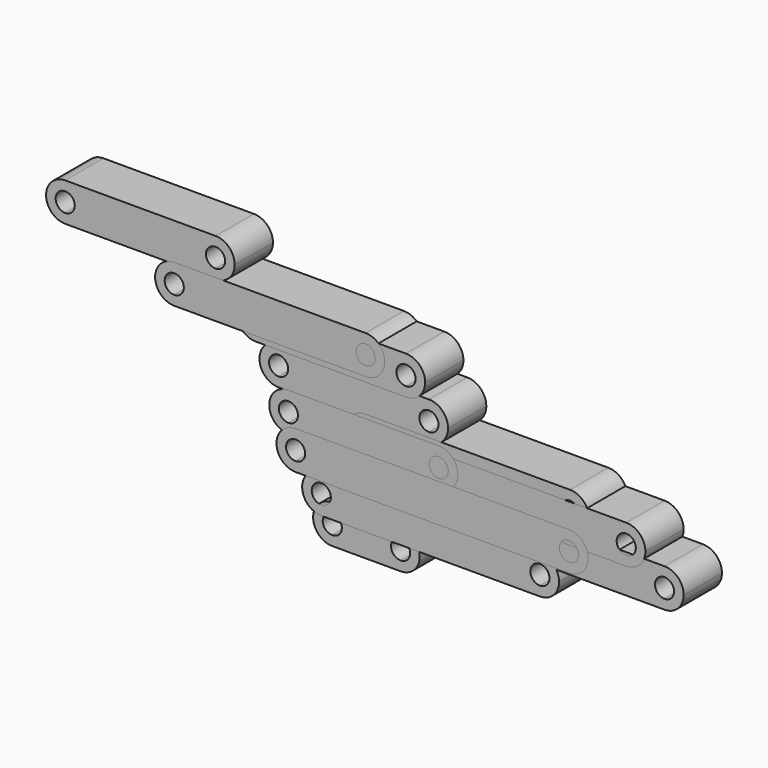
from build123d import *

# Parameters (mm, degrees)
F2_DEPTH  = 6.35
F4_DEPTH  = 6.35
F6_DEPTH  = 6.35
F8_DEPTH  = 6.35
F10_DEPTH = 6.35
F12_DEPTH = 6.35
F14_DEPTH = 6.35
F16_DEPTH = 6.35
F18_DEPTH = 6.35
F20_DEPTH = 6.35
F22_DEPTH = 6.35
F24_DEPTH = 6.35


# Not quite as in the source:
# - a variable given as a bare number and used for a length is read in inches; the dataset says mm whatever the document's units were


with BuildPart() as f2:
    # F1 (on Front) → F2 (new body)
    with BuildSketch(Plane.XZ):
        with BuildLine():
            ThreePointArc((-20.3833308847, 1.27), (-19.4853052726, 0.8980256121), (-19.1133308847, 0))
            ThreePointArc((-19.1133308847, 0), (-19.4853052726, -0.8980256121), (-20.3833308847, -1.27))
            Line((-20.3833308847, -1.27), (-20.3833308847, -2.54))
            ThreePointArc((-20.3833308847, -2.54), (-18.5872796605, -1.7960512242), (-17.8433308847, 0))
            ThreePointArc((-17.8433308847, 0), (-18.5872796605, 1.7960512242), (-20.3833308847, 2.54))
            Line((-20.3833308847, 2.54), (-20.3833308847, 1.27))
        make_face()
        with BuildLine():
            ThreePointArc((-20.3833308847, -1.27), (-21.6533308847, 0), (-20.3833308847, 1.27))
            Line((-20.3833308847, 1.27), (-20.3833308847, 2.54))
            ThreePointArc((-20.3833308847, 2.54), (-22.9233308847, 0), (-20.3833308847, -2.54))
            Line((-20.3833308847, -2.54), (-20.3833308847, -1.27))
        make_face()
        with BuildLine():
            Line((3.202383401, 2.54), (-20.3833308847, 2.54))
            ThreePointArc((-20.3833308847, 2.54), (-18.5872796605, 1.7960512242), (-17.8433308847, 0))
            ThreePointArc((-17.8433308847, 0), (-18.5872796605, -1.7960512242), (-20.3833308847, -2.54))
            Line((-20.3833308847, -2.54), (3.202383401, -2.54))
            ThreePointArc((3.202383401, -2.54), (0.662383401, 0), (3.202383401, 2.54))
        make_face()
        with BuildLine():
            Line((3.202383401, 1.27), (3.202383401, 2.54))
            ThreePointArc((3.202383401, 2.54), (0.662383401, 0), (3.202383401, -2.54))
            Line((3.202383401, -2.54), (3.202383401, -1.27))
            ThreePointArc((3.202383401, -1.27), (1.932383401, 0), (3.202383401, 1.27))
        make_face()
        with BuildLine():
            ThreePointArc((5.742383401, 0), (4.9984346253, 1.7960512242), (3.202383401, 2.54))
            Line((3.202383401, 2.54), (3.202383401, 1.27))
            ThreePointArc((3.202383401, 1.27), (4.1004090131, 0.8980256121), (4.472383401, 0))
            ThreePointArc((4.472383401, 0), (4.1004090131, -0.8980256121), (3.202383401, -1.27))
            Line((3.202383401, -1.27), (3.202383401, -2.54))
            ThreePointArc((3.202383401, -2.54), (4.9984346253, -1.7960512242), (5.742383401, 0))
        make_face()
    extrude(amount=F2_DEPTH)


with BuildPart() as f4:
    # F3 (on Front) → F4 (new body)
    with BuildSketch(Plane.XZ):
        with BuildLine():
            ThreePointArc((-40.9096366516, -5.6361554968), (-40.0116110395, -6.0081298847), (-39.6396366516, -6.9061554968))
            ThreePointArc((-39.6396366516, -6.9061554968), (-40.0116110395, -7.8041811089), (-40.9096366516, -8.1761554968))
            Line((-40.9096366516, -8.1761554968), (-40.9096366516, -9.4461554968))
            ThreePointArc((-40.9096366516, -9.4461554968), (-39.1135854274, -8.702206721), (-38.3696366516, -6.9061554968))
            ThreePointArc((-38.3696366516, -6.9061554968), (-39.1135854274, -5.1101042726), (-40.9096366516, -4.3661554968))
            Line((-40.9096366516, -4.3661554968), (-40.9096366516, -5.6361554968))
        make_face()
        with BuildLine():
            ThreePointArc((-40.9096366516, -8.1761554968), (-42.1796366516, -6.9061554968), (-40.9096366516, -5.6361554968))
            Line((-40.9096366516, -5.6361554968), (-40.9096366516, -4.3661554968))
            ThreePointArc((-40.9096366516, -4.3661554968), (-43.4496366516, -6.9061554968), (-40.9096366516, -9.4461554968))
            Line((-40.9096366516, -9.4461554968), (-40.9096366516, -8.1761554968))
        make_face()
        with BuildLine():
            Line((-31.8382080802, -4.3661554968), (-40.9096366516, -4.3661554968))
            ThreePointArc((-40.9096366516, -4.3661554968), (-39.1135854274, -5.1101042726), (-38.3696366516, -6.9061554968))
            ThreePointArc((-38.3696366516, -6.9061554968), (-39.1135854274, -8.702206721), (-40.9096366516, -9.4461554968))
            Line((-40.9096366516, -9.4461554968), (-31.8382080802, -9.4461554968))
            ThreePointArc((-31.8382080802, -9.4461554968), (-34.3782080802, -6.9061554968), (-31.8382080802, -4.3661554968))
        make_face()
        with BuildLine():
            Line((-31.8382080802, -5.6361554968), (-31.8382080802, -4.3661554968))
            ThreePointArc((-31.8382080802, -4.3661554968), (-34.3782080802, -6.9061554968), (-31.8382080802, -9.4461554968))
            Line((-31.8382080802, -9.4461554968), (-31.8382080802, -8.1761554968))
            ThreePointArc((-31.8382080802, -8.1761554968), (-33.1082080802, -6.9061554968), (-31.8382080802, -5.6361554968))
        make_face()
        with BuildLine():
            ThreePointArc((-29.2982080802, -6.9061554968), (-30.042156856, -5.1101042726), (-31.8382080802, -4.3661554968))
            Line((-31.8382080802, -4.3661554968), (-31.8382080802, -5.6361554968))
            ThreePointArc((-31.8382080802, -5.6361554968), (-30.9401824681, -6.0081298847), (-30.5682080802, -6.9061554968))
            ThreePointArc((-30.5682080802, -6.9061554968), (-30.9401824681, -7.8041811089), (-31.8382080802, -8.1761554968))
            Line((-31.8382080802, -8.1761554968), (-31.8382080802, -9.4461554968))
            ThreePointArc((-31.8382080802, -9.4461554968), (-30.042156856, -8.702206721), (-29.2982080802, -6.9061554968))
        make_face()
    extrude(amount=F4_DEPTH)


with BuildPart() as f6:
    # F5 (on Front) → F6 (new body)
    with BuildSketch(Plane.XZ):
        with BuildLine():
            ThreePointArc((-42.3683448485, -2.56121497), (-41.4703192364, -2.9331893579), (-41.0983448485, -3.83121497))
            ThreePointArc((-41.0983448485, -3.83121497), (-41.4703192364, -4.7292405821), (-42.3683448485, -5.10121497))
            Line((-42.3683448485, -5.10121497), (-42.3683448485, -6.37121497))
            ThreePointArc((-42.3683448485, -6.37121497), (-40.5722936243, -5.6272661942), (-39.8283448485, -3.83121497))
            ThreePointArc((-39.8283448485, -3.83121497), (-40.5722936243, -2.0351637458), (-42.3683448485, -1.29121497))
            Line((-42.3683448485, -1.29121497), (-42.3683448485, -2.56121497))
        make_face()
        with BuildLine():
            ThreePointArc((-42.3683448485, -5.10121497), (-43.6383448485, -3.83121497), (-42.3683448485, -2.56121497))
            Line((-42.3683448485, -2.56121497), (-42.3683448485, -1.29121497))
            ThreePointArc((-42.3683448485, -1.29121497), (-44.9083448485, -3.83121497), (-42.3683448485, -6.37121497))
            Line((-42.3683448485, -6.37121497), (-42.3683448485, -5.10121497))
        make_face()
        with BuildLine():
            Line((-13.3397734199, -1.29121497), (-42.3683448485, -1.29121497))
            ThreePointArc((-42.3683448485, -1.29121497), (-40.5722936243, -2.0351637458), (-39.8283448485, -3.83121497))
            ThreePointArc((-39.8283448485, -3.83121497), (-40.5722936243, -5.6272661942), (-42.3683448485, -6.37121497))
            Line((-42.3683448485, -6.37121497), (-13.3397734199, -6.37121497))
            ThreePointArc((-13.3397734199, -6.37121497), (-15.8797734199, -3.83121497), (-13.3397734199, -1.29121497))
        make_face()
        with BuildLine():
            Line((-13.3397734199, -2.56121497), (-13.3397734199, -1.29121497))
            ThreePointArc((-13.3397734199, -1.29121497), (-15.8797734199, -3.83121497), (-13.3397734199, -6.37121497))
            Line((-13.3397734199, -6.37121497), (-13.3397734199, -5.10121497))
            ThreePointArc((-13.3397734199, -5.10121497), (-14.6097734199, -3.83121497), (-13.3397734199, -2.56121497))
        make_face()
        with BuildLine():
            ThreePointArc((-10.7997734199, -3.83121497), (-11.5437221957, -2.0351637458), (-13.3397734199, -1.29121497))
            Line((-13.3397734199, -1.29121497), (-13.3397734199, -2.56121497))
            ThreePointArc((-13.3397734199, -2.56121497), (-12.4417478078, -2.9331893579), (-12.0697734199, -3.83121497))
            ThreePointArc((-12.0697734199, -3.83121497), (-12.4417478078, -4.7292405821), (-13.3397734199, -5.10121497))
            Line((-13.3397734199, -5.10121497), (-13.3397734199, -6.37121497))
            ThreePointArc((-13.3397734199, -6.37121497), (-11.5437221957, -5.6272661942), (-10.7997734199, -3.83121497))
        make_face()
    extrude(amount=F6_DEPTH)


with BuildPart() as f8:
    # F7 (on Front) → F8 (new body)
    with BuildSketch(Plane.XZ):
        with BuildLine():
            ThreePointArc((-48.0340662203, 10.5945822936), (-47.1360406082, 10.2226079057), (-46.7640662203, 9.3245822936))
            ThreePointArc((-46.7640662203, 9.3245822936), (-47.1360406082, 8.4265566815), (-48.0340662203, 8.0545822936))
            Line((-48.0340662203, 8.0545822936), (-48.0340662203, 6.7845822936))
            ThreePointArc((-48.0340662203, 6.7845822936), (-46.2380149961, 7.5285310694), (-45.4940662203, 9.3245822936))
            ThreePointArc((-45.4940662203, 9.3245822936), (-46.2380149961, 11.1206335178), (-48.0340662203, 11.8645822936))
            Line((-48.0340662203, 11.8645822936), (-48.0340662203, 10.5945822936))
        make_face()
        with BuildLine():
            ThreePointArc((-48.0340662203, 8.0545822936), (-49.3040662203, 9.3245822936), (-48.0340662203, 10.5945822936))
            Line((-48.0340662203, 10.5945822936), (-48.0340662203, 11.8645822936))
            ThreePointArc((-48.0340662203, 11.8645822936), (-50.5740662203, 9.3245822936), (-48.0340662203, 6.7845822936))
            Line((-48.0340662203, 6.7845822936), (-48.0340662203, 8.0545822936))
        make_face()
        with BuildLine():
            Line((-28.0769233631, 11.8645822936), (-48.0340662203, 11.8645822936))
            ThreePointArc((-48.0340662203, 11.8645822936), (-46.2380149961, 11.1206335178), (-45.4940662203, 9.3245822936))
            ThreePointArc((-45.4940662203, 9.3245822936), (-46.2380149961, 7.5285310694), (-48.0340662203, 6.7845822936))
            Line((-48.0340662203, 6.7845822936), (-28.0769233631, 6.7845822936))
            ThreePointArc((-28.0769233631, 6.7845822936), (-30.6169233631, 9.3245822936), (-28.0769233631, 11.8645822936))
        make_face()
        with BuildLine():
            Line((-28.0769233631, 10.5945822936), (-28.0769233631, 11.8645822936))
            ThreePointArc((-28.0769233631, 11.8645822936), (-30.6169233631, 9.3245822936), (-28.0769233631, 6.7845822936))
            Line((-28.0769233631, 6.7845822936), (-28.0769233631, 8.0545822936))
            ThreePointArc((-28.0769233631, 8.0545822936), (-29.3469233631, 9.3245822936), (-28.0769233631, 10.5945822936))
        make_face()
        with BuildLine():
            ThreePointArc((-25.5369233631, 9.3245822936), (-26.2808721389, 11.1206335178), (-28.0769233631, 11.8645822936))
            Line((-28.0769233631, 11.8645822936), (-28.0769233631, 10.5945822936))
            ThreePointArc((-28.0769233631, 10.5945822936), (-27.178897751, 10.2226079057), (-26.8069233631, 9.3245822936))
            ThreePointArc((-26.8069233631, 9.3245822936), (-27.178897751, 8.4265566815), (-28.0769233631, 8.0545822936))
            Line((-28.0769233631, 8.0545822936), (-28.0769233631, 6.7845822936))
            ThreePointArc((-28.0769233631, 6.7845822936), (-26.2808721389, 7.5285310694), (-25.5369233631, 9.3245822936))
        make_face()
    extrude(amount=F8_DEPTH)


with BuildPart() as f10:
    # F9 (on Front) → F10 (new body)
    with BuildSketch(Plane.XZ):
        with BuildLine():
            ThreePointArc((-38.6977585754, 1.7656836929), (-37.7997329633, 1.393709305), (-37.4277585754, 0.4956836929))
            ThreePointArc((-37.4277585754, 0.4956836929), (-37.7997329633, -0.4023419192), (-38.6977585754, -0.7743163071))
            Line((-38.6977585754, -0.7743163071), (-38.6977585754, -2.0443163071))
            ThreePointArc((-38.6977585754, -2.0443163071), (-36.9017073512, -1.3003675314), (-36.1577585754, 0.4956836929))
            ThreePointArc((-36.1577585754, 0.4956836929), (-36.9017073512, 2.2917349171), (-38.6977585754, 3.0356836929))
            Line((-38.6977585754, 3.0356836929), (-38.6977585754, 1.7656836929))
        make_face()
        with BuildLine():
            ThreePointArc((-38.6977585754, -0.7743163071), (-39.9677585754, 0.4956836929), (-38.6977585754, 1.7656836929))
            Line((-38.6977585754, 1.7656836929), (-38.6977585754, 3.0356836929))
            ThreePointArc((-38.6977585754, 3.0356836929), (-41.2377585754, 0.4956836929), (-38.6977585754, -2.0443163071))
            Line((-38.6977585754, -2.0443163071), (-38.6977585754, -0.7743163071))
        make_face()
        with BuildLine():
            Line((-18.7406157183, 3.0356836929), (-38.6977585754, 3.0356836929))
            ThreePointArc((-38.6977585754, 3.0356836929), (-36.9017073512, 2.2917349171), (-36.1577585754, 0.4956836929))
            ThreePointArc((-36.1577585754, 0.4956836929), (-36.9017073512, -1.3003675314), (-38.6977585754, -2.0443163071))
            Line((-38.6977585754, -2.0443163071), (-18.7406157183, -2.0443163071))
            ThreePointArc((-18.7406157183, -2.0443163071), (-21.2806157183, 0.4956836929), (-18.7406157183, 3.0356836929))
        make_face()
        with BuildLine():
            Line((-18.7406157183, 1.7656836929), (-18.7406157183, 3.0356836929))
            ThreePointArc((-18.7406157183, 3.0356836929), (-21.2806157183, 0.4956836929), (-18.7406157183, -2.0443163071))
            Line((-18.7406157183, -2.0443163071), (-18.7406157183, -0.7743163071))
            ThreePointArc((-18.7406157183, -0.7743163071), (-20.0106157183, 0.4956836929), (-18.7406157183, 1.7656836929))
        make_face()
        with BuildLine():
            ThreePointArc((-16.2006157183, 0.4956836929), (-16.9445644941, 2.2917349171), (-18.7406157183, 3.0356836929))
            Line((-18.7406157183, 3.0356836929), (-18.7406157183, 1.7656836929))
            ThreePointArc((-18.7406157183, 1.7656836929), (-17.8425901062, 1.393709305), (-17.4706157183, 0.4956836929))
            ThreePointArc((-17.4706157183, 0.4956836929), (-17.8425901062, -0.4023419192), (-18.7406157183, -0.7743163071))
            Line((-18.7406157183, -0.7743163071), (-18.7406157183, -2.0443163071))
            ThreePointArc((-18.7406157183, -2.0443163071), (-16.9445644941, -1.3003675314), (-16.2006157183, 0.4956836929))
        make_face()
    extrude(amount=F10_DEPTH)


with BuildPart() as f12:
    # F11 (on Front) → F12 (new body)
    with BuildSketch(Plane.XZ):
        with BuildLine():
            ThreePointArc((-36.5666438616, 6.1293925312), (-35.6686182495, 5.7574181433), (-35.2966438616, 4.8593925312))
            ThreePointArc((-35.2966438616, 4.8593925312), (-35.6686182495, 3.9613669191), (-36.5666438616, 3.5893925312))
            Line((-36.5666438616, 3.5893925312), (-36.5666438616, 2.3193925312))
            ThreePointArc((-36.5666438616, 2.3193925312), (-34.7705926374, 3.063341307), (-34.0266438616, 4.8593925312))
            ThreePointArc((-34.0266438616, 4.8593925312), (-34.7705926374, 6.6554437554), (-36.5666438616, 7.3993925312))
            Line((-36.5666438616, 7.3993925312), (-36.5666438616, 6.1293925312))
        make_face()
        with BuildLine():
            ThreePointArc((-36.5666438616, 3.5893925312), (-37.8366438616, 4.8593925312), (-36.5666438616, 6.1293925312))
            Line((-36.5666438616, 6.1293925312), (-36.5666438616, 7.3993925312))
            ThreePointArc((-36.5666438616, 7.3993925312), (-39.1066438616, 4.8593925312), (-36.5666438616, 2.3193925312))
            Line((-36.5666438616, 2.3193925312), (-36.5666438616, 3.5893925312))
        make_face()
        with BuildLine():
            Line((-9.3523581473, 7.3993925312), (-36.5666438616, 7.3993925312))
            ThreePointArc((-36.5666438616, 7.3993925312), (-34.7705926374, 6.6554437554), (-34.0266438616, 4.8593925312))
            ThreePointArc((-34.0266438616, 4.8593925312), (-34.7705926374, 3.063341307), (-36.5666438616, 2.3193925312))
            Line((-36.5666438616, 2.3193925312), (-9.3523581473, 2.3193925312))
            ThreePointArc((-9.3523581473, 2.3193925312), (-11.8923581473, 4.8593925312), (-9.3523581473, 7.3993925312))
        make_face()
        with BuildLine():
            Line((-9.3523581473, 6.1293925312), (-9.3523581473, 7.3993925312))
            ThreePointArc((-9.3523581473, 7.3993925312), (-11.8923581473, 4.8593925312), (-9.3523581473, 2.3193925312))
            Line((-9.3523581473, 2.3193925312), (-9.3523581473, 3.5893925312))
            ThreePointArc((-9.3523581473, 3.5893925312), (-10.6223581473, 4.8593925312), (-9.3523581473, 6.1293925312))
        make_face()
        with BuildLine():
            ThreePointArc((-6.8123581473, 4.8593925312), (-7.5563069231, 6.6554437554), (-9.3523581473, 7.3993925312))
            Line((-9.3523581473, 7.3993925312), (-9.3523581473, 6.1293925312))
            ThreePointArc((-9.3523581473, 6.1293925312), (-8.4543325352, 5.7574181433), (-8.0823581473, 4.8593925312))
            ThreePointArc((-8.0823581473, 4.8593925312), (-8.4543325352, 3.9613669191), (-9.3523581473, 3.5893925312))
            Line((-9.3523581473, 3.5893925312), (-9.3523581473, 2.3193925312))
            ThreePointArc((-9.3523581473, 2.3193925312), (-7.5563069231, 3.063341307), (-6.8123581473, 4.8593925312))
        make_face()
    extrude(amount=F12_DEPTH)


with BuildPart() as f14:
    # F13 (on Front) → F14 (new body)
    with BuildSketch(Plane.XZ):
        with BuildLine():
            ThreePointArc((-34.5370125747, 4.7086499319), (-33.6389869626, 4.336675544), (-33.2670125747, 3.4386499319))
            ThreePointArc((-33.2670125747, 3.4386499319), (-33.6389869626, 2.5406243198), (-34.5370125747, 2.1686499319))
            Line((-34.5370125747, 2.1686499319), (-34.5370125747, 0.8986499319))
            ThreePointArc((-34.5370125747, 0.8986499319), (-32.7409613505, 1.6425987077), (-31.9970125747, 3.4386499319))
            ThreePointArc((-31.9970125747, 3.4386499319), (-32.7409613505, 5.2347011561), (-34.5370125747, 5.9786499319))
            Line((-34.5370125747, 5.9786499319), (-34.5370125747, 4.7086499319))
        make_face()
        with BuildLine():
            ThreePointArc((-34.5370125747, 2.1686499319), (-35.8070125747, 3.4386499319), (-34.5370125747, 4.7086499319))
            Line((-34.5370125747, 4.7086499319), (-34.5370125747, 5.9786499319))
            ThreePointArc((-34.5370125747, 5.9786499319), (-37.0770125747, 3.4386499319), (-34.5370125747, 0.8986499319))
            Line((-34.5370125747, 0.8986499319), (-34.5370125747, 2.1686499319))
        make_face()
        with BuildLine():
            Line((-1.8798697176, 5.9786499319), (-34.5370125747, 5.9786499319))
            ThreePointArc((-34.5370125747, 5.9786499319), (-32.7409613505, 5.2347011561), (-31.9970125747, 3.4386499319))
            ThreePointArc((-31.9970125747, 3.4386499319), (-32.7409613505, 1.6425987077), (-34.5370125747, 0.8986499319))
            Line((-34.5370125747, 0.8986499319), (-1.8798697176, 0.8986499319))
            ThreePointArc((-1.8798697176, 0.8986499319), (-4.4198697176, 3.4386499319), (-1.8798697176, 5.9786499319))
        make_face()
        with BuildLine():
            Line((-1.8798697176, 4.7086499319), (-1.8798697176, 5.9786499319))
            ThreePointArc((-1.8798697176, 5.9786499319), (-4.4198697176, 3.4386499319), (-1.8798697176, 0.8986499319))
            Line((-1.8798697176, 0.8986499319), (-1.8798697176, 2.1686499319))
            ThreePointArc((-1.8798697176, 2.1686499319), (-3.1498697176, 3.4386499319), (-1.8798697176, 4.7086499319))
        make_face()
        with BuildLine():
            ThreePointArc((0.6601302824, 3.4386499319), (-0.0838184934, 5.2347011561), (-1.8798697176, 5.9786499319))
            Line((-1.8798697176, 5.9786499319), (-1.8798697176, 4.7086499319))
            ThreePointArc((-1.8798697176, 4.7086499319), (-0.9818441055, 4.336675544), (-0.6098697176, 3.4386499319))
            ThreePointArc((-0.6098697176, 3.4386499319), (-0.9818441055, 2.5406243198), (-1.8798697176, 2.1686499319))
            Line((-1.8798697176, 2.1686499319), (-1.8798697176, 0.8986499319))
            ThreePointArc((-1.8798697176, 0.8986499319), (-0.0838184934, 1.6425987077), (0.6601302824, 3.4386499319))
        make_face()
    extrude(amount=F14_DEPTH)


with BuildPart() as f16:
    # F15 (on Front) → F16 (new body)
    with BuildSketch(Plane.XZ):
        with BuildLine():
            ThreePointArc((-51.0785131506, 14.958291423), (-50.1804875384, 14.5863170351), (-49.8085131506, 13.688291423))
            ThreePointArc((-49.8085131506, 13.688291423), (-50.1804875384, 12.7902658109), (-51.0785131506, 12.418291423))
            Line((-51.0785131506, 12.418291423), (-51.0785131506, 11.148291423))
            ThreePointArc((-51.0785131506, 11.148291423), (-49.2824619263, 11.8922401988), (-48.5385131506, 13.688291423))
            ThreePointArc((-48.5385131506, 13.688291423), (-49.2824619263, 15.4843426472), (-51.0785131506, 16.228291423))
            Line((-51.0785131506, 16.228291423), (-51.0785131506, 14.958291423))
        make_face()
        with BuildLine():
            ThreePointArc((-51.0785131506, 12.418291423), (-52.3485131506, 13.688291423), (-51.0785131506, 14.958291423))
            Line((-51.0785131506, 14.958291423), (-51.0785131506, 16.228291423))
            ThreePointArc((-51.0785131506, 16.228291423), (-53.6185131506, 13.688291423), (-51.0785131506, 11.148291423))
            Line((-51.0785131506, 11.148291423), (-51.0785131506, 12.418291423))
        make_face()
        with BuildLine():
            Line((-31.1213702934, 16.228291423), (-51.0785131506, 16.228291423))
            ThreePointArc((-51.0785131506, 16.228291423), (-49.2824619263, 15.4843426472), (-48.5385131506, 13.688291423))
            ThreePointArc((-48.5385131506, 13.688291423), (-49.2824619263, 11.8922401988), (-51.0785131506, 11.148291423))
            Line((-51.0785131506, 11.148291423), (-31.1213702934, 11.148291423))
            ThreePointArc((-31.1213702934, 11.148291423), (-33.6613702934, 13.688291423), (-31.1213702934, 16.228291423))
        make_face()
        with BuildLine():
            Line((-31.1213702934, 14.958291423), (-31.1213702934, 16.228291423))
            ThreePointArc((-31.1213702934, 16.228291423), (-33.6613702934, 13.688291423), (-31.1213702934, 11.148291423))
            Line((-31.1213702934, 11.148291423), (-31.1213702934, 12.418291423))
            ThreePointArc((-31.1213702934, 12.418291423), (-32.3913702934, 13.688291423), (-31.1213702934, 14.958291423))
        make_face()
        with BuildLine():
            ThreePointArc((-28.5813702934, 13.688291423), (-29.3253190692, 15.4843426472), (-31.1213702934, 16.228291423))
            Line((-31.1213702934, 16.228291423), (-31.1213702934, 14.958291423))
            ThreePointArc((-31.1213702934, 14.958291423), (-30.2233446813, 14.5863170351), (-29.8513702934, 13.688291423))
            ThreePointArc((-29.8513702934, 13.688291423), (-30.2233446813, 12.7902658109), (-31.1213702934, 12.418291423))
            Line((-31.1213702934, 12.418291423), (-31.1213702934, 11.148291423))
            ThreePointArc((-31.1213702934, 11.148291423), (-29.3253190692, 11.8922401988), (-28.5813702934, 13.688291423))
        make_face()
    extrude(amount=F16_DEPTH)


with BuildPart() as f18:
    # F17 (on Front) → F18 (new body)
    with BuildSketch(Plane.XZ):
        with BuildLine():
            ThreePointArc((-76.3660705439, 20.4931088877), (-75.4680449318, 20.1211344998), (-75.0960705439, 19.2231088877))
            ThreePointArc((-75.0960705439, 19.2231088877), (-75.4680449318, 18.3250832756), (-76.3660705439, 17.9531088877))
            Line((-76.3660705439, 17.9531088877), (-76.3660705439, 16.6831088877))
            ThreePointArc((-76.3660705439, 16.6831088877), (-74.5700193197, 17.4270576635), (-73.8260705439, 19.2231088877))
            ThreePointArc((-73.8260705439, 19.2231088877), (-74.5700193197, 21.0191601119), (-76.3660705439, 21.7631088877))
            Line((-76.3660705439, 21.7631088877), (-76.3660705439, 20.4931088877))
        make_face()
        with BuildLine():
            ThreePointArc((-76.3660705439, 17.9531088877), (-77.6360705439, 19.2231088877), (-76.3660705439, 20.4931088877))
            Line((-76.3660705439, 20.4931088877), (-76.3660705439, 21.7631088877))
            ThreePointArc((-76.3660705439, 21.7631088877), (-78.9060705439, 19.2231088877), (-76.3660705439, 16.6831088877))
            Line((-76.3660705439, 16.6831088877), (-76.3660705439, 17.9531088877))
        make_face()
        with BuildLine():
            Line((-56.4089276867, 21.7631088877), (-76.3660705439, 21.7631088877))
            ThreePointArc((-76.3660705439, 21.7631088877), (-74.5700193197, 21.0191601119), (-73.8260705439, 19.2231088877))
            ThreePointArc((-73.8260705439, 19.2231088877), (-74.5700193197, 17.4270576635), (-76.3660705439, 16.6831088877))
            Line((-76.3660705439, 16.6831088877), (-56.4089276867, 16.6831088877))
            ThreePointArc((-56.4089276867, 16.6831088877), (-58.9489276867, 19.2231088877), (-56.4089276867, 21.7631088877))
        make_face()
        with BuildLine():
            Line((-56.4089276867, 20.4931088877), (-56.4089276867, 21.7631088877))
            ThreePointArc((-56.4089276867, 21.7631088877), (-58.9489276867, 19.2231088877), (-56.4089276867, 16.6831088877))
            Line((-56.4089276867, 16.6831088877), (-56.4089276867, 17.9531088877))
            ThreePointArc((-56.4089276867, 17.9531088877), (-57.6789276867, 19.2231088877), (-56.4089276867, 20.4931088877))
        make_face()
        with BuildLine():
            ThreePointArc((-53.8689276867, 19.2231088877), (-54.6128764625, 21.0191601119), (-56.4089276867, 21.7631088877))
            Line((-56.4089276867, 21.7631088877), (-56.4089276867, 20.4931088877))
            ThreePointArc((-56.4089276867, 20.4931088877), (-55.5109020746, 20.1211344998), (-55.1389276867, 19.2231088877))
            ThreePointArc((-55.1389276867, 19.2231088877), (-55.5109020746, 18.3250832756), (-56.4089276867, 17.9531088877))
            Line((-56.4089276867, 17.9531088877), (-56.4089276867, 16.6831088877))
            ThreePointArc((-56.4089276867, 16.6831088877), (-54.6128764625, 17.4270576635), (-53.8689276867, 19.2231088877))
        make_face()
    extrude(amount=F18_DEPTH)


with BuildPart() as f20:
    # F19 (on Front) → F20 (new body)
    with BuildSketch(Plane.XZ):
        with BuildLine():
            ThreePointArc((-46.7356982431, 5.5978406374), (-45.837672631, 5.2258662495), (-45.4656982431, 4.3278406374))
            ThreePointArc((-45.4656982431, 4.3278406374), (-45.837672631, 3.4298150253), (-46.7356982431, 3.0578406374))
            Line((-46.7356982431, 3.0578406374), (-46.7356982431, 1.7878406374))
            ThreePointArc((-46.7356982431, 1.7878406374), (-44.9396470189, 2.5317894132), (-44.1956982431, 4.3278406374))
            ThreePointArc((-44.1956982431, 4.3278406374), (-44.9396470189, 6.1238918616), (-46.7356982431, 6.8678406374))
            Line((-46.7356982431, 6.8678406374), (-46.7356982431, 5.5978406374))
        make_face()
        with BuildLine():
            ThreePointArc((-46.7356982431, 3.0578406374), (-48.0056982431, 4.3278406374), (-46.7356982431, 5.5978406374))
            Line((-46.7356982431, 5.5978406374), (-46.7356982431, 6.8678406374))
            ThreePointArc((-46.7356982431, 6.8678406374), (-49.2756982431, 4.3278406374), (-46.7356982431, 1.7878406374))
            Line((-46.7356982431, 1.7878406374), (-46.7356982431, 3.0578406374))
        make_face()
        with BuildLine():
            Line((-26.778555386, 6.8678406374), (-46.7356982431, 6.8678406374))
            ThreePointArc((-46.7356982431, 6.8678406374), (-44.9396470189, 6.1238918616), (-44.1956982431, 4.3278406374))
            ThreePointArc((-44.1956982431, 4.3278406374), (-44.9396470189, 2.5317894132), (-46.7356982431, 1.7878406374))
            Line((-46.7356982431, 1.7878406374), (-26.778555386, 1.7878406374))
            ThreePointArc((-26.778555386, 1.7878406374), (-29.318555386, 4.3278406374), (-26.778555386, 6.8678406374))
        make_face()
        with BuildLine():
            Line((-26.778555386, 5.5978406374), (-26.778555386, 6.8678406374))
            ThreePointArc((-26.778555386, 6.8678406374), (-29.318555386, 4.3278406374), (-26.778555386, 1.7878406374))
            Line((-26.778555386, 1.7878406374), (-26.778555386, 3.0578406374))
            ThreePointArc((-26.778555386, 3.0578406374), (-28.048555386, 4.3278406374), (-26.778555386, 5.5978406374))
        make_face()
        with BuildLine():
            ThreePointArc((-24.238555386, 4.3278406374), (-24.9825041618, 6.1238918616), (-26.778555386, 6.8678406374))
            Line((-26.778555386, 6.8678406374), (-26.778555386, 5.5978406374))
            ThreePointArc((-26.778555386, 5.5978406374), (-25.8805297739, 5.2258662495), (-25.508555386, 4.3278406374))
            ThreePointArc((-25.508555386, 4.3278406374), (-25.8805297739, 3.4298150253), (-26.778555386, 3.0578406374))
            Line((-26.778555386, 3.0578406374), (-26.778555386, 1.7878406374))
            ThreePointArc((-26.778555386, 1.7878406374), (-24.9825041618, 2.5317894132), (-24.238555386, 4.3278406374))
        make_face()
    extrude(amount=F20_DEPTH)


with BuildPart() as f22:
    # F21 (on Front) → F22 (new body)
    with BuildSketch(Plane.XZ):
        with BuildLine():
            ThreePointArc((-45.7747111819, 1.4335720691), (-44.8766855698, 1.0615976812), (-44.5047111819, 0.1635720691))
            ThreePointArc((-44.5047111819, 0.1635720691), (-44.8766855698, -0.734453543), (-45.7747111819, -1.1064279309))
            Line((-45.7747111819, -1.1064279309), (-45.7747111819, -2.3764279309))
            ThreePointArc((-45.7747111819, -2.3764279309), (-43.9786599576, -1.6324791551), (-43.2347111819, 0.1635720691))
            ThreePointArc((-43.2347111819, 0.1635720691), (-43.9786599576, 1.9596232934), (-45.7747111819, 2.7035720691))
            Line((-45.7747111819, 2.7035720691), (-45.7747111819, 1.4335720691))
        make_face()
        with BuildLine():
            ThreePointArc((-45.7747111819, -1.1064279309), (-47.0447111819, 0.1635720691), (-45.7747111819, 1.4335720691))
            Line((-45.7747111819, 1.4335720691), (-45.7747111819, 2.7035720691))
            ThreePointArc((-45.7747111819, 2.7035720691), (-48.3147111819, 0.1635720691), (-45.7747111819, -2.3764279309))
            Line((-45.7747111819, -2.3764279309), (-45.7747111819, -1.1064279309))
        make_face()
        with BuildLine():
            Line((-9.4889968961, 2.7035720691), (-45.7747111819, 2.7035720691))
            ThreePointArc((-45.7747111819, 2.7035720691), (-43.9786599576, 1.9596232934), (-43.2347111819, 0.1635720691))
            ThreePointArc((-43.2347111819, 0.1635720691), (-43.9786599576, -1.6324791551), (-45.7747111819, -2.3764279309))
            Line((-45.7747111819, -2.3764279309), (-9.4889968961, -2.3764279309))
            ThreePointArc((-9.4889968961, -2.3764279309), (-12.0289968961, 0.1635720691), (-9.4889968961, 2.7035720691))
        make_face()
        with BuildLine():
            Line((-9.4889968961, 1.4335720691), (-9.4889968961, 2.7035720691))
            ThreePointArc((-9.4889968961, 2.7035720691), (-12.0289968961, 0.1635720691), (-9.4889968961, -2.3764279309))
            Line((-9.4889968961, -2.3764279309), (-9.4889968961, -1.1064279309))
            ThreePointArc((-9.4889968961, -1.1064279309), (-10.7589968961, 0.1635720691), (-9.4889968961, 1.4335720691))
        make_face()
        with BuildLine():
            ThreePointArc((-6.9489968961, 0.1635720691), (-7.6929456719, 1.9596232934), (-9.4889968961, 2.7035720691))
            Line((-9.4889968961, 2.7035720691), (-9.4889968961, 1.4335720691))
            ThreePointArc((-9.4889968961, 1.4335720691), (-8.590971284, 1.0615976812), (-8.2189968961, 0.1635720691))
            ThreePointArc((-8.2189968961, 0.1635720691), (-8.590971284, -0.734453543), (-9.4889968961, -1.1064279309))
            Line((-9.4889968961, -1.1064279309), (-9.4889968961, -2.3764279309))
            ThreePointArc((-9.4889968961, -2.3764279309), (-7.6929456719, -1.6324791551), (-6.9489968961, 0.1635720691))
        make_face()
    extrude(amount=F22_DEPTH)


with BuildPart() as f24:
    # F23 (on Front) → F24 (new body)
    with BuildSketch(Plane.XZ):
        with BuildLine():
            ThreePointArc((-61.8885717145, 15.6220319834), (-60.9905461024, 15.2500575955), (-60.6185717145, 14.3520319834))
            ThreePointArc((-60.6185717145, 14.3520319834), (-60.9905461024, 13.4540063713), (-61.8885717145, 13.0820319834))
            Line((-61.8885717145, 13.0820319834), (-61.8885717145, 11.8120319834))
            ThreePointArc((-61.8885717145, 11.8120319834), (-60.0925204903, 12.5559807592), (-59.3485717145, 14.3520319834))
            ThreePointArc((-59.3485717145, 14.3520319834), (-60.0925204903, 16.1480832076), (-61.8885717145, 16.8920319834))
            Line((-61.8885717145, 16.8920319834), (-61.8885717145, 15.6220319834))
        make_face()
        with BuildLine():
            ThreePointArc((-61.8885717145, 13.0820319834), (-63.1585717145, 14.3520319834), (-61.8885717145, 15.6220319834))
            Line((-61.8885717145, 15.6220319834), (-61.8885717145, 16.8920319834))
            ThreePointArc((-61.8885717145, 16.8920319834), (-64.4285717145, 14.3520319834), (-61.8885717145, 11.8120319834))
            Line((-61.8885717145, 11.8120319834), (-61.8885717145, 13.0820319834))
        make_face()
        with BuildLine():
            Line((-36.4885717145, 16.8920319834), (-61.8885717145, 16.8920319834))
            ThreePointArc((-61.8885717145, 16.8920319834), (-60.0925204903, 16.1480832076), (-59.3485717145, 14.3520319834))
            ThreePointArc((-59.3485717145, 14.3520319834), (-60.0925204903, 12.5559807592), (-61.8885717145, 11.8120319834))
            Line((-61.8885717145, 11.8120319834), (-36.4885717145, 11.8120319834))
            ThreePointArc((-36.4885717145, 11.8120319834), (-39.0285717145, 14.3520319834), (-36.4885717145, 16.8920319834))
        make_face()
        with BuildLine():
            Line((-36.4885717145, 15.6220319834), (-36.4885717145, 16.8920319834))
            ThreePointArc((-36.4885717145, 16.8920319834), (-39.0285717145, 14.3520319834), (-36.4885717145, 11.8120319834))
            Line((-36.4885717145, 11.8120319834), (-36.4885717145, 13.0820319834))
            ThreePointArc((-36.4885717145, 13.0820319834), (-37.7585717145, 14.3520319834), (-36.4885717145, 15.6220319834))
        make_face()
        with BuildLine():
            ThreePointArc((-33.9485717145, 14.3520319834), (-34.6925204903, 16.1480832076), (-36.4885717145, 16.8920319834))
            Line((-36.4885717145, 16.8920319834), (-36.4885717145, 15.6220319834))
            ThreePointArc((-36.4885717145, 15.6220319834), (-35.5905461024, 15.2500575955), (-35.2185717145, 14.3520319834))
            ThreePointArc((-35.2185717145, 14.3520319834), (-35.5905461024, 13.4540063713), (-36.4885717145, 13.0820319834))
            Line((-36.4885717145, 13.0820319834), (-36.4885717145, 11.8120319834))
            ThreePointArc((-36.4885717145, 11.8120319834), (-34.6925204903, 12.5559807592), (-33.9485717145, 14.3520319834))
        make_face()
    extrude(amount=F24_DEPTH)


solid = Compound([f2.part, f4.part, f6.part, f8.part, f10.part, f12.part, f14.part, f16.part, f18.part, f20.part, f22.part, f24.part])
